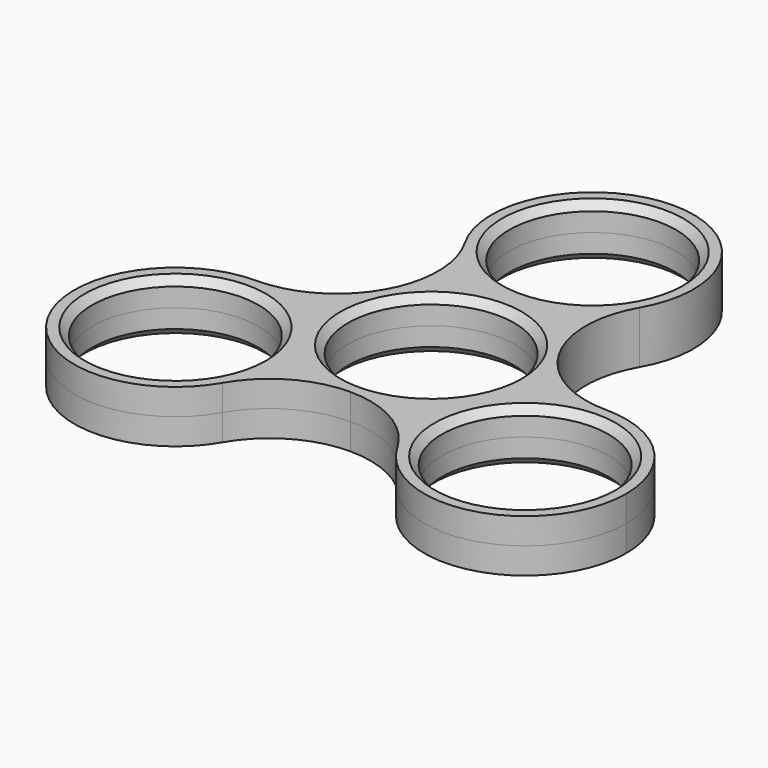
from build123d import *

# Parameters (mm, degrees)
F0_R     = 11.125
F1_DEPTH = 3.5
F2_SIZE  = 1
F3_SIZE  = 1


# Not quite as in the source:
# - a feature names something its author has since deleted; it is built from what else it names


with BuildPart() as f1:
    # F0 (on Top) → F1 (new body, symmetric)
    with BuildSketch(Plane.XY):
        with BuildLine():
            ThreePointArc((-1.36e-08, 13.5), (6.7500001307, 11.6913428757), (11.6913431087, 6.7499997269))
            ThreePointArc((11.6913431087, 6.7499997269), (9.8826859022, 13.4999998423), (11.6913429511, 20.25))
            ThreePointArc((11.6913429511, 20.25), (6.7499999941, 15.3086570455), (-1.36e-08, 13.5))
        make_face()
        with BuildLine():
            ThreePointArc((-11.691342964, 6.7499999776), (-6.7500000171, 11.6913429412), (-1.36e-08, 13.5))
            ThreePointArc((-1.36e-08, 13.5), (-6.7500000059, 15.3086570523), (-11.6913429511, 20.25))
            ThreePointArc((-11.6913429511, 20.25), (-9.8826859022, 13.4999999871), (-11.691342964, 6.7499999776))
        make_face()
        with BuildLine():
            ThreePointArc((-11.6913429875, -6.749999937), (-13.5, 2.34e-08), (-11.691342964, 6.7499999776))
            ThreePointArc((-11.691342964, 6.7499999776), (-16.6326859134, 1.8086570424), (-23.3826859022, 0))
            ThreePointArc((-23.3826859022, 0), (-16.6326859337, -1.8086570307), (-11.6913429875, -6.749999937))
        make_face()
        with BuildLine():
            ThreePointArc((-11.6913429511, -20.25), (-6.7500000035, -15.3086570509), (-8.1e-09, -13.5))
            ThreePointArc((-8.1e-09, -13.5), (-6.750000035, -11.6913429309), (-11.6913429875, -6.749999937))
            ThreePointArc((-11.6913429875, -6.749999937), (-10.3426872567, -10.005942856), (-9.8826859022, -13.5))
            ThreePointArc((-9.8826859022, -13.5), (-10.3426872473, -16.9940571089), (-11.6913429511, -20.25))
        make_face()
        with BuildLine():
            ThreePointArc((11.6913429511, -20.25), (9.8826859022, -13.5000001869), (11.6913427641, -6.7500003238))
            ThreePointArc((11.6913427641, -6.7500003238), (6.7499998346, -11.6913430466), (-8.1e-09, -13.5))
            ThreePointArc((-8.1e-09, -13.5), (6.7499999965, -15.3086570469), (11.6913429511, -20.25))
        make_face()
        with BuildLine():
            ThreePointArc((11.6913431087, 6.7499997269), (13.0399986957, 3.4940569566), (13.5, 0))
            ThreePointArc((13.5, 0), (13.0399986065, -3.4940572895), (11.6913427641, -6.7500003238))
            ThreePointArc((11.6913427641, -6.7500003238), (16.6326857403, -1.8086571424), (23.3826859022, 0))
            ThreePointArc((23.3826859022, 0), (16.6326860387, 1.8086569701), (11.6913431087, 6.7499997269))
        make_face()
        with BuildLine():
            ThreePointArc((11.6913427641, -6.7500003238), (13.0399986065, -3.4940572895), (13.5, 0))
            ThreePointArc((13.5, 0), (13.0399986957, 3.4940569566), (11.6913431087, 6.7499997269))
            ThreePointArc((11.6913431087, 6.7499997269), (6.7500001307, 11.6913428757), (-1.36e-08, 13.5))
            ThreePointArc((-1.36e-08, 13.5), (-6.7500000171, 11.6913429412), (-11.691342964, 6.7499999776))
            ThreePointArc((-11.691342964, 6.7499999776), (-13.5, 2.34e-08), (-11.6913429875, -6.749999937))
            ThreePointArc((-11.6913429875, -6.749999937), (-6.750000035, -11.6913429309), (-8.1e-09, -13.5))
            ThreePointArc((-8.1e-09, -13.5), (6.7499998346, -11.6913430466), (11.6913427641, -6.7500003238))
        make_face()
        Circle(F0_R, mode=Mode.SUBTRACT)
        with BuildLine():
            ThreePointArc((-11.6913429511, 20.25), (-6.7500000059, 15.3086570523), (-1.36e-08, 13.5))
            ThreePointArc((-1.36e-08, 13.5), (6.7499999941, 15.3086570455), (11.6913429511, 20.25))
            ThreePointArc((11.6913429511, 20.25), (13.0399986549, 23.5059428911), (13.5, 27))
            ThreePointArc((13.5, 27), (-3.4940571089, 40.0399986549), (-11.6913429511, 20.25))
        make_face()
        with Locations((0, 27)):
            Circle(F0_R, mode=Mode.SUBTRACT)
        with BuildLine():
            ThreePointArc((-9.8826859022, -13.5), (-10.3426872567, -10.005942856), (-11.6913429875, -6.749999937))
            ThreePointArc((-11.6913429875, -6.749999937), (-16.6326859337, -1.8086570307), (-23.3826859022, 0))
            ThreePointArc((-23.3826859022, 0), (-35.0740288533, -20.25), (-11.6913429511, -20.25))
            ThreePointArc((-11.6913429511, -20.25), (-10.3426872473, -16.9940571089), (-9.8826859022, -13.5))
        make_face()
        with Locations((-23.3826859022, -13.5)):
            Circle(F0_R, mode=Mode.SUBTRACT)
        with BuildLine():
            ThreePointArc((23.3826859022, 0), (16.6326857403, -1.8086571424), (11.6913427641, -6.7500003238))
            ThreePointArc((11.6913427641, -6.7500003238), (9.8826859022, -13.5000001869), (11.6913429511, -20.25))
            ThreePointArc((11.6913429511, -20.25), (26.8767430111, -26.5399986549), (36.8826859022, -13.5))
            ThreePointArc((36.8826859022, -13.5), (32.9286274482, -3.954058454), (23.3826859022, 0))
        make_face()
        with Locations((23.3826859022, -13.5)):
            Circle(F0_R, mode=Mode.SUBTRACT)
    extrude(amount=F1_DEPTH, both=True)

    # F2
    f2_edges = [f1.edges().sort_by_distance(p)[0] for p in [
        (-11.125, 0, 3.5),
        (-11.125, 27, 3.5),
        (-34.507686, -13.5, 3.5),
        (12.257686, -13.5, 3.5),
    ]]
    chamfer(f2_edges, length=F2_SIZE)

    # F3
    f3_edges = [f1.edges().sort_by_distance(p)[0] for p in [
        (-11.125, 0, -3.5),
        (-11.125, 27, -3.5),
        (-34.507686, -13.5, -3.5),
        (12.257686, -13.5, -3.5),
    ]]
    chamfer(f3_edges, length=F3_SIZE)


solid = f1.part
